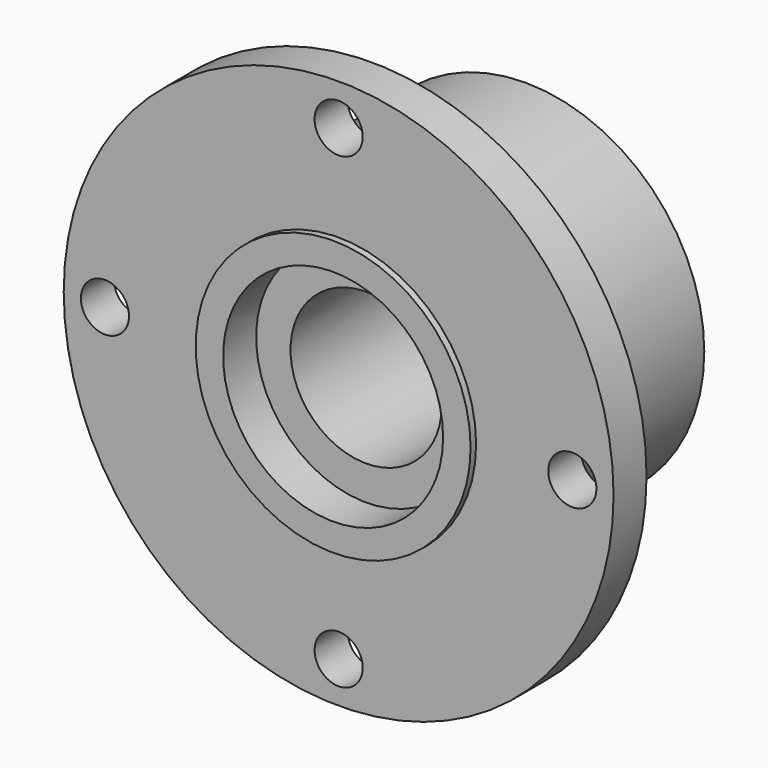
from build123d import *

# Parameters (mm, degrees)
F0_R             = 63.5
F1_DEPTH         = 9.525
F2_R             = 31.75
F3_DEPTH         = 1.5875
F4_R             = 25.4
F5_DEPTH         = 9.525
F6_R             = 41.275
F7_DEPTH         = 44.45
F8_R             = 17.4625
F9_DEPTH         = 55.5635
F10_R            = 5.55625
F11_DEPTH        = 53.976
F11_COPIES_COUNT = 4


# Not quite as in the source:
# - a pattern or mirror of a feature is missing from the dataset's text; its kind, count and spacing are read off the source's solid


with BuildPart() as f1:
    # F0 (on Front) → F1 (new body)
    with BuildSketch(Plane.XZ):
        Circle(F0_R)
    extrude(amount=-F1_DEPTH)

    # F2 (on face) → F3 (join)
    with BuildSketch(Plane.XZ):
        Circle(F2_R)
    extrude(amount=F3_DEPTH)

    # F4 (on face) → F5 (cut)
    with BuildSketch(Plane.XZ.offset(1.5875)):
        Circle(F4_R)
    extrude(amount=-F5_DEPTH, mode=Mode.SUBTRACT)

    # F6 (on face) → F7 (join)
    with BuildSketch(Plane(origin=(0, 9.525, 0), x_dir=(-1, 0, 0), z_dir=(0, 1, 0))):
        Circle(F6_R)
    extrude(amount=F7_DEPTH)

    # F8 (on face) → F9 (cut, through all)
    with BuildSketch(Plane.XZ.offset(1.5875)):
        Circle(F8_R)
    extrude(amount=-F9_DEPTH, mode=Mode.SUBTRACT)

    # F10 (on face) → F11 (cut, through all)
    with BuildSketch(Plane.XZ):
        with Locations((53.975, 0)):
            Circle(F10_R)
    f11 = extrude(amount=-F11_DEPTH, mode=Mode.SUBTRACT)

    # F11_copies: F11 ×4 about axis
    f11_copies_axis = Axis((0, 0, 0), (0, 1, 0))
    for i in range(1, F11_COPIES_COUNT):
        add(f11.rotate(f11_copies_axis, i * 360 / F11_COPIES_COUNT), mode=Mode.SUBTRACT)


solid = f1.part
